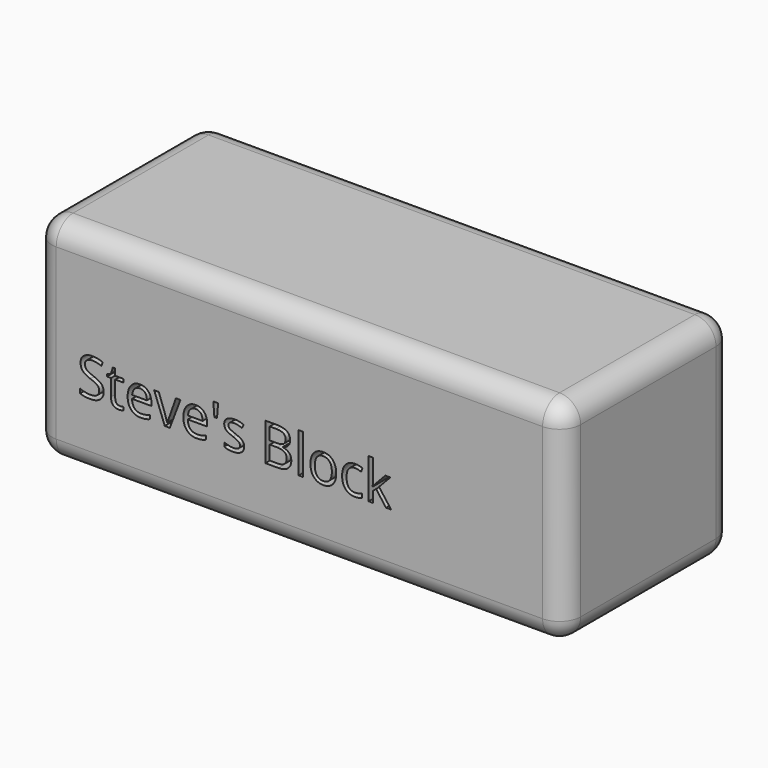
from build123d import *

# Parameters (mm, degrees)
F0_W         = 127
F0_H         = 50.8
F1_DEPTH     = 50.8
F2_R         = 5.08
F3_TEXT_SIZE = 12.6090441348
F4_DEPTH     = 25.4


# Not quite as in the source:
# - Text() gives the source's letters only with a copy of the font that has no kerning and outlines rounded to 1/6400 em; it was checked with that copy


with BuildPart() as f1:
    # F0 (on Top) → F1 (new body)
    with BuildSketch(Plane.XY):
        with Locations((5.4233763367, 6.0917460924)):
            Rectangle(F0_W, F0_H)
    extrude(amount=F1_DEPTH)

    # F2
    f2_edges = [f1.edges().sort_by_distance(p)[0] for p in [
        (68.923376, 6.091746, 50.8),
        (5.423376, 31.491746, 50.8),
        (-58.076624, 6.091746, 50.8),
        (5.423376, -19.308254, 50.8),
        (68.923376, -19.308254, 25.4),
        (68.923376, 31.491746, 25.4),
        (68.923376, 6.091746, 0),
        (-58.076624, 31.491746, 25.4),
        (-58.076624, -19.308254, 25.4),
        (-58.076624, 6.091746, 0),
        (5.423376, 31.491746, 0),
        (5.423376, -19.308254, 0),
    ]]
    fillet(f2_edges, radius=F2_R)

    # F3 (on face) → F4 (cut)
    with BuildSketch(Plane.XZ.offset(19.3082539076)):
        with Locations((-47.9166236633, 16.321488223)):
            Text("Steve's Block", F3_TEXT_SIZE, font='Open Sans', text_align=(TextAlign.LEFT, TextAlign.BOTTOM))
    extrude(amount=-F4_DEPTH, mode=Mode.SUBTRACT)


solid = f1.part
